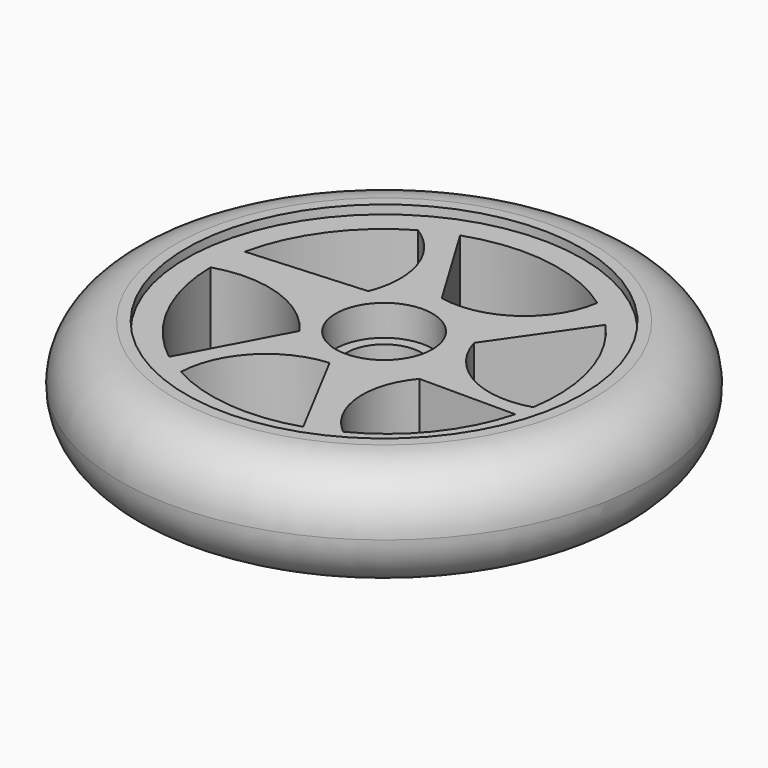
from build123d import *

# Parameters (mm, degrees)
F0_R      = 60
F1_DEPTH  = 25
F2_R      = 45
F3_DEPTH  = 2
F4_R      = 11
F5_DEPTH  = 7
F6_R      = 45
F7_DEPTH  = 2
F8_R      = 11
F9_DEPTH  = 7
F10_R     = 8.5
F11_DEPTH = 25
F12_R     = 12.49999
F16_DEPTH = 25


# Not quite as in the source:
# - a fillet or chamfer is up to 0.001 mm smaller than in the source, because OpenCascade refuses the exact size


with BuildPart() as f1:
    # F0 (on Top) → F1 (new body)
    with BuildSketch(Plane.XY):
        Circle(F0_R)
    extrude(amount=F1_DEPTH)

    # F2 (on face) → F3 (cut)
    with BuildSketch(Plane.XY.offset(25)):
        Circle(F2_R)
    extrude(amount=-F3_DEPTH, mode=Mode.SUBTRACT)

    # F4 (on face) → F5 (cut)
    with BuildSketch(Plane.XY.offset(23)):
        Circle(F4_R)
    extrude(amount=-F5_DEPTH, mode=Mode.SUBTRACT)

    # F6 (on face) → F7 (cut)
    with BuildSketch(Plane(origin=(0, 0, 0), x_dir=(1, 0, 0), z_dir=(0, 0, -1))):
        Circle(F6_R)
    extrude(amount=-F7_DEPTH, mode=Mode.SUBTRACT)

    # F8 (on face) → F9 (cut)
    with BuildSketch(Plane(origin=(0, 0, 2), x_dir=(1, 0, 0), z_dir=(0, 0, -1))):
        Circle(F8_R)
    extrude(amount=-F9_DEPTH, mode=Mode.SUBTRACT)

    # F10 (on face) → F11 (cut)
    with BuildSketch(Plane(origin=(0, 0, 9), x_dir=(1, 0, 0), z_dir=(0, 0, -1))):
        Circle(F10_R)
    extrude(amount=-F11_DEPTH, mode=Mode.SUBTRACT)

    # F12 (radius 12.5 in the source; OpenCascade refuses exactly that, so slightly less here)
    f12_edges = [f1.edges().sort_by_distance(p)[0] for p in [
        (-60, 0, 25),
        (-60, 0, 0),
    ]]
    fillet(f12_edges, radius=F12_R)

    # F15 (on face) → F16 (cut)
    with BuildSketch(Plane.XY.offset(23)):
        with BuildLine():
            Line((-23.7309150398, -31.4583554864), (-11.8406927213, -9.2094279826))
            ThreePointArc((-11.8406927213, -9.2094279826), (-24.1709240611, -0.1529805421), (-39.4689776003, 0))
            ThreePointArc((-39.4689776003, 0), (-35.1668885168, -17.5136562569), (-23.7309150398, -31.4583554864))
        make_face()
        with BuildLine():
            Line((11.6958646104, -37.6011095941), (0, -15.4828215018))
            ThreePointArc((0, -15.4828215018), (-12.8825559704, -21.5513966495), (-18.4614025056, -34.6534699202))
            ThreePointArc((-18.4614025056, -34.6534699202), (-3.6886632813, -39.2568911162), (11.6958646104, -37.6011095941))
        make_face()
        with BuildLine():
            Line((38.0679219961, -10.3157823905), (16.2651948631, -10.3157823905))
            ThreePointArc((16.2651948631, -10.3157823905), (12.2364949642, -22.929504934), (18.3915793896, -34.6534699202))
            ThreePointArc((18.3915793896, -34.6534699202), (30.8515845586, -24.6043058224), (38.0679219961, -10.3157823905))
        make_face()
        with BuildLine():
            Line((29.1008390486, 26.5384856611), (15.2093013749, 6.5587405115))
            ThreePointArc((15.2093013749, 6.5587405115), (24.360120091, -4.7843640185), (38.8653166592, -6.1995587312))
            ThreePointArc((38.8653166592, -6.1995587312), (37.7282086233, 11.2864894274), (29.1008390486, 26.5384856611))
        make_face()
        with BuildLine():
            Line((-12.5216757879, 37.253908813), (0, 16.3887739182))
            ThreePointArc((0, 16.3887739182), (14.7450774696, 19.4214078257), (22.6965453476, 32.2037525475))
            ThreePointArc((22.6965453476, 32.2037525475), (5.7090018341, 39.0634462479), (-12.5216757879, 37.253908813))
        make_face()
        with BuildLine():
            Line((-38.4788028896, 8.5062459111), (-11.8609527126, 10.3406049311))
            ThreePointArc((-11.8609527126, 10.3406049311), (-11.4093820553, 23.6626254803), (-19.6125917137, 34.1691710055))
            ThreePointArc((-19.6125917137, 34.1691710055), (-31.7739639836, 23.3434055945), (-38.4788028896, 8.5062459111))
        make_face()
    extrude(amount=-F16_DEPTH, mode=Mode.SUBTRACT)


solid = f1.part
